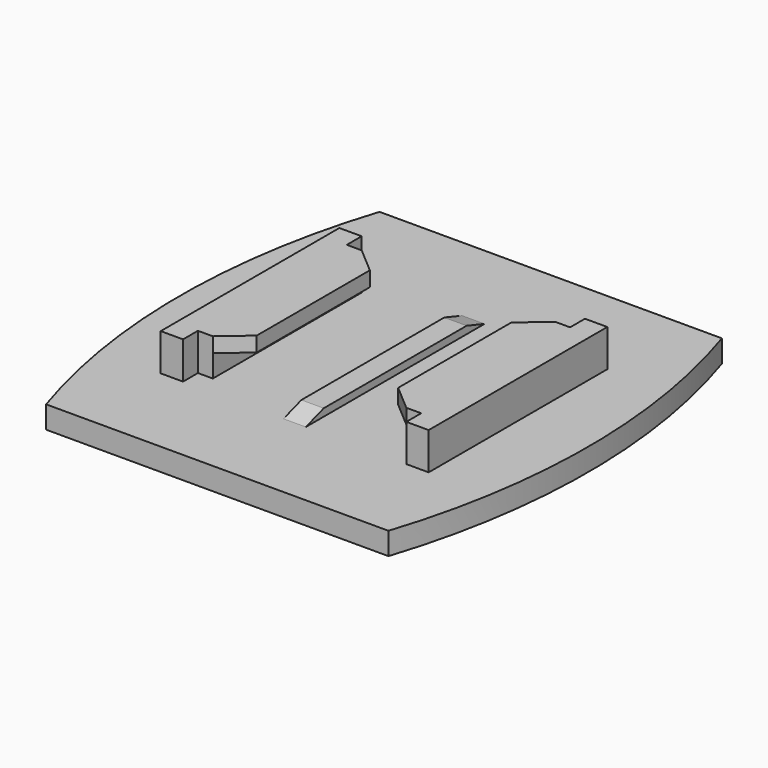
from build123d import *

# Parameters (mm, degrees)
F1_DEPTH    = 3
F3_DEPTH    = 3
F5_DEPTH    = 2
F7_DEPTH    = 2
F8_W        = 3
F8_H        = 30
F9_DEPTH    = 1
F10_SIZE2   = 2.99999
F10_SIZE    = 0.99999
F10_2_SIZE2 = 2.99999
F10_2_SIZE  = 0.99999


# Not quite as in the source:
# - a fillet or chamfer is up to 0.001 mm smaller than in the source, because OpenCascade refuses the exact size


with BuildPart() as f1:
    # F0 (on Top) → F1 (new body)
    with BuildSketch(Plane.XY):
        with BuildLine():
            ThreePointArc((0, -56), (4.4433524368, -28), (0, 0))
            Line((0, 0), (-46, 0))
            ThreePointArc((-46, 0), (-50.4433524368, -28), (-46, -56))
            Line((-46, -56), (0, -56))
        make_face()
    extrude(amount=F1_DEPTH)

    # F2 (on face) → F3 (join)
    with BuildSketch(Plane.XY.offset(3)):
        Polygon((-38, -13), (-41, -13), (-41, -43), (-38, -43), (-38, -40.5), (-36, -40.5), (-36, -15.5), (-38, -15.5), align=None)
        Polygon((-5, -43), (-5, -13), (-8, -13), (-8, -15.5), (-10, -15.5), (-10, -40.5), (-8, -40.5), (-8, -43), align=None)
    extrude(amount=F3_DEPTH)

    # F4 (on face) → F5 (join)
    with BuildSketch(Plane.XY.offset(6)):
        Polygon((-38, -13), (-41, -13), (-41, -43), (-38, -43), (-38, -40.5), (-36, -40.5), (-32.5, -37.5), (-32.5, -18.5), (-36, -15.5), (-38, -15.5), align=None)
    extrude(amount=F5_DEPTH)

    # F6 (on face) → F7 (join)
    with BuildSketch(Plane.XY.offset(6)):
        Polygon((-5, -13), (-8, -13), (-8, -15.5), (-10, -15.5), (-13.5, -18.5), (-13.5, -37.5), (-10, -40.5), (-8, -40.5), (-8, -43), (-5, -43), align=None)
    extrude(amount=F7_DEPTH)

    # F8 (on face) → F9 (join)
    with BuildSketch(Plane.XY.offset(3)):
        with Locations((-23, -28)):
            Rectangle(F8_W, F8_H)
    extrude(amount=F9_DEPTH)

    # F10 (size 1 and 3 in the source; OpenCascade refuses exactly that, so slightly less here)
    f10_edges = [f1.edges().sort_by_distance(p)[0] for p in [
        (-23, -13, 4),
    ]]
    f10_side = f1.faces().sort_by_distance((-23, -13, 3.5))[0]
    chamfer(f10_edges, length=F10_SIZE, length2=F10_SIZE2, reference=f10_side)

    # F10#2 (size 1 and 3 in the source; OpenCascade refuses exactly that, so slightly less here)
    f10_2_edges = [f1.edges().sort_by_distance(p)[0] for p in [
        (-23, -43, 4),
    ]]
    f10_2_side = f1.faces().sort_by_distance((-23, -43, 3.5))[0]
    chamfer(f10_2_edges, length=F10_2_SIZE, length2=F10_2_SIZE2, reference=f10_2_side)


solid = f1.part
